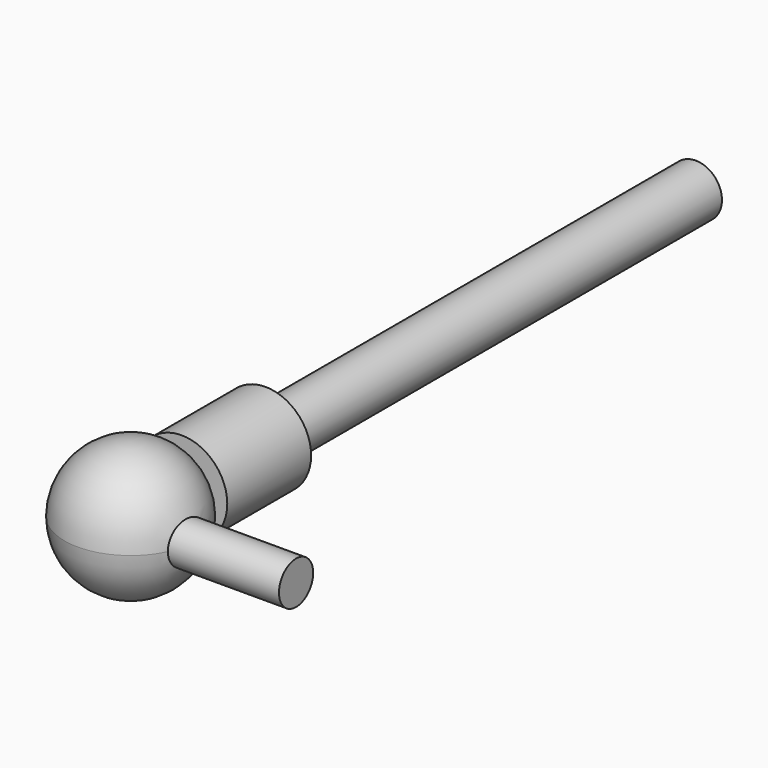
from build123d import *

# Parameters (mm, degrees)
F0_R     = 5.08
F1_DEPTH = 11.684
F4_R     = 2.921
F5_DEPTH = 59.944
F6_R     = 2.38125
F7_DEPTH = 19.05


with BuildPart() as f1:
    # F0 (on Front) → F1 (new body)
    with BuildSketch(Plane.XZ):
        Circle(F0_R)
    extrude(amount=F1_DEPTH)

    # F2 (on Right) → F3 (revolve)
    with BuildSketch(Plane.YZ):
        with BuildLine():
            ThreePointArc((-18.796, -7.366), (-13.5874514498, -5.2085485502), (-11.43, 0))
            ThreePointArc((-11.43, 0), (-13.5874514498, 5.2085485502), (-18.796, 7.366))
            Line((-18.796, 7.366), (-18.796, 0))
            Line((-18.796, 0), (-18.796, -7.366))
        make_face()
    revolve(axis=Axis((0, -18.796, 0), (0, 0, -1)))

    # F4 (on face) → F5 (join)
    with BuildSketch(Plane(origin=(0, 0, 0), x_dir=(-1, 0, 0), z_dir=(0, 1, 0))):
        Circle(F4_R)
    extrude(amount=F5_DEPTH)

    # F6 (on Right) → F7 (join)
    with BuildSketch(Plane.YZ):
        with Locations((-19.558, 0)):
            Circle(F6_R)
    extrude(amount=F7_DEPTH)


solid = f1.part
